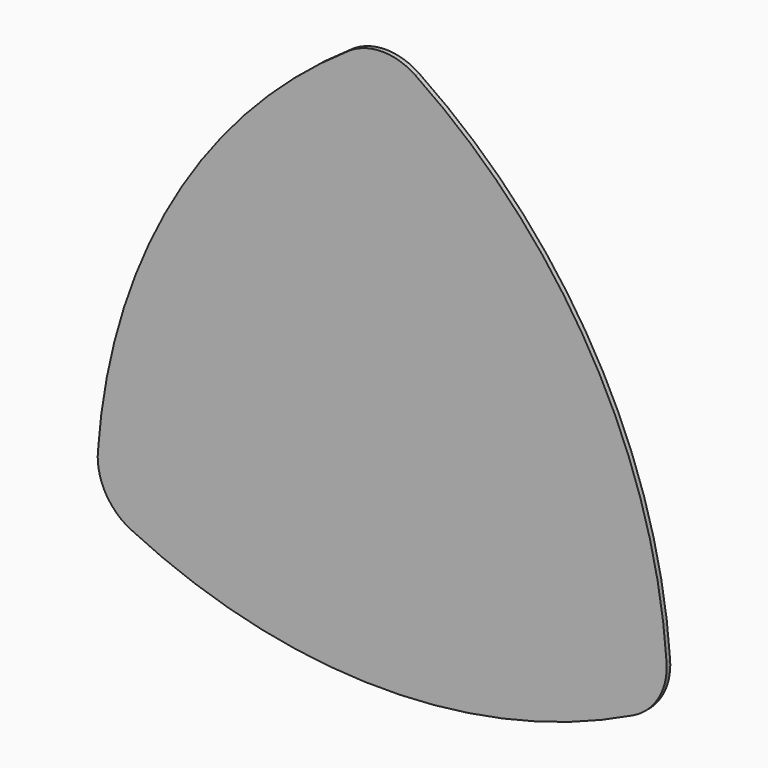
from build123d import *

# Parameters (mm, degrees)
F1_DEPTH = 9.525
F2_R     = 127


with BuildPart() as f1:
    # F0 (on Front) → F1 (new body)
    with BuildSketch(Plane.XZ):
        with BuildLine():
            ThreePointArc((-609.6, 0), (0, -163.341827706), (609.6, 0))
            ThreePointArc((609.6, 0), (446.258172294, 609.6), (0, 1055.858172294))
            ThreePointArc((0, 1055.858172294), (-446.258172294, 609.6), (-609.6, 0))
        make_face()
    extrude(amount=F1_DEPTH)

    # F2
    f2_edges = [f1.edges().sort_by_distance(p)[0] for p in [
        (0, -4.7625, 1055.858172),
        (-609.6, -4.7625, 0),
        (609.6, -4.7625, 0),
    ]]
    fillet(f2_edges, radius=F2_R)


solid = f1.part
